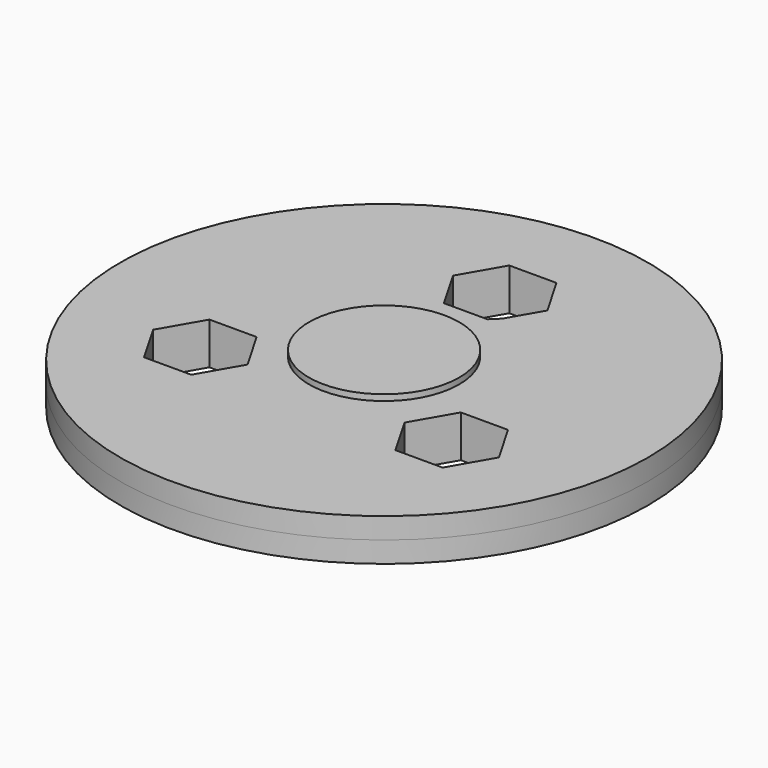
from build123d import *

# Parameters (mm, degrees)
F0_R           = 12.5
F0_R_2         = 11.1
F1_DEPTH       = 1.5
F2_DEPTH       = 3.5
F0_R_3         = 4
F3_DEPTH       = 3.5
F4_START       = 3.5
F0_R_4         = 7.5
F4_DEPTH       = 0.5
F5_START       = 4
F5_DEPTH       = 1
F8_R           = 2.5702688947
F8_R_2         = 2.6203971893
F8_R_3         = 1.9967906643
F8_R_4         = 1.9017675277
F9_DEPTH       = 0.25
F7_TEXT_SIZE   = 4.6829839388
F10_DEPTH      = 0.25
F12_DEPTH      = 3.5
F12_DEPTH_BACK = 3.5
F14_DEPTH      = 3.5
F14_DEPTH_BACK = 3.5
F16_DEPTH      = 3.5
F16_DEPTH_BACK = 3.5
F17_R          = 70.1541780483
F17_R_2        = 43.9177935103
F18_DEPTH      = 25
F18_DEPTH_BACK = 25


# Not quite as in the source:
# - Text() gives the source's letters only with a copy of the font that has no kerning and outlines rounded to 1/6400 em; it was checked with that copy


with BuildPart() as f1:
    # F0 (on Top) → F1 (new body, symmetric)
    with BuildSketch(Plane.XY):
        with BuildLine():
            ThreePointArc((-3.1128243989, 13.7521025397), (-7.595688921, 11.879204932), (-11.1767513589, 8.5959425929))
            ThreePointArc((-11.1767513589, 8.5959425929), (-12.2109581934, 7.05), (-13.0326803344, 5.3813793122))
            ThreePointArc((-13.0326803344, 5.3813793122), (-14.0855377083, 0.6384570988), (-13.4660823543, -4.1802662628))
            ThreePointArc((-13.4660823543, -4.1802662628), (-17.4115804876, -1.8023831124), (-21.9880010034, -1.2754494733))
            ThreePointArc((-21.9880010034, -1.2754494733), (-30.3108891325, -17.5), (-12.0985721468, -18.4044427108))
            ThreePointArc((-12.0985721468, -18.4044427108), (-10.2666998065, -14.1776794661), (-10.3532579553, -9.5718362768))
            ThreePointArc((-10.3532579553, -9.5718362768), (-6.4898487874, -12.5176620308), (-1.8559289755, -13.9773219051))
            ThreePointArc((-1.8559289755, -13.9773219051), (0, -14.1), (1.8559289755, -13.9773219051))
            ThreePointArc((1.8559289755, -13.9773219051), (6.4898487874, -12.5176620308), (10.3532579553, -9.5718362768))
            ThreePointArc((10.3532579553, -9.5718362768), (10.2666998065, -14.1776794661), (12.0985721468, -18.4044427108))
            ThreePointArc((12.0985721468, -18.4044427108), (30.3108891325, -17.5), (21.9880010034, -1.2754494733))
            ThreePointArc((21.9880010034, -1.2754494733), (17.4115804876, -1.8023831124), (13.4660823543, -4.1802662628))
            ThreePointArc((13.4660823543, -4.1802662628), (14.0855377083, 0.6384570988), (13.0326803344, 5.3813793122))
            ThreePointArc((13.0326803344, 5.3813793122), (12.2109581934, 7.05), (11.1767513589, 8.5959425929))
            ThreePointArc((11.1767513589, 8.5959425929), (7.595688921, 11.879204932), (3.1128243989, 13.7521025397))
            ThreePointArc((3.1128243989, 13.7521025397), (7.1448806811, 15.9800625785), (9.8894288566, 19.6798921841))
            ThreePointArc((9.8894288566, 19.6798921841), (0, 35), (-9.8894288566, 19.6798921841))
            ThreePointArc((-9.8894288566, 19.6798921841), (-7.1448806811, 15.9800625785), (-3.1128243989, 13.7521025397))
        make_face()
        Polygon((-16.9868310906, -5.2740181695), (-13.0608492601, -12.0740181695), (-16.9868310906, -18.8740181695), (-24.8387947516, -18.8740181695), (-28.7647765821, -12.0740181695), (-24.8387947516, -5.2740181695), align=None, mode=Mode.SUBTRACT)
        Circle(F0_R, mode=Mode.SUBTRACT)
        Polygon((13.0608492601, -12.0740181695), (16.9868310906, -5.2740181695), (24.8387947516, -5.2740181695), (28.7647765821, -12.0740181695), (24.8387947516, -18.8740181695), (16.9868310906, -18.8740181695), align=None, mode=Mode.SUBTRACT)
        Polygon((7.851963661, 24.148036339), (3.9259818305, 17.348036339), (-3.9259818305, 17.348036339), (-7.851963661, 24.148036339), (-3.9259818305, 30.948036339), (3.9259818305, 30.948036339), align=None, mode=Mode.SUBTRACT)
        Circle(F0_R)
        Circle(F0_R_2, mode=Mode.SUBTRACT)
        with BuildLine():
            ThreePointArc((-13.4660823543, -4.1802662628), (-14.0855377083, 0.6384570988), (-13.0326803344, 5.3813793122))
            ThreePointArc((-13.0326803344, 5.3813793122), (-16.589205157, 0.8137766881), (-21.9880010034, -1.2754494733))
            ThreePointArc((-21.9880010034, -1.2754494733), (-17.4115804876, -1.8023831124), (-13.4660823543, -4.1802662628))
        make_face()
        with BuildLine():
            ThreePointArc((-9.8894288566, 19.6798921841), (-8.9993538634, 13.9597847505), (-11.1767513589, 8.5959425929))
            ThreePointArc((-11.1767513589, 8.5959425929), (-7.595688921, 11.879204932), (-3.1128243989, 13.7521025397))
            ThreePointArc((-3.1128243989, 13.7521025397), (-7.1448806811, 15.9800625785), (-9.8894288566, 19.6798921841))
        make_face()
        with BuildLine():
            ThreePointArc((-10.3532579553, -9.5718362768), (-10.2666998065, -14.1776794661), (-12.0985721468, -18.4044427108))
            ThreePointArc((-12.0985721468, -18.4044427108), (-7.5898512936, -14.7735614386), (-1.8559289755, -13.9773219051))
            ThreePointArc((-1.8559289755, -13.9773219051), (-6.4898487874, -12.5176620308), (-10.3532579553, -9.5718362768))
        make_face()
        with BuildLine():
            ThreePointArc((21.9880010034, -1.2754494733), (16.589205157, 0.8137766881), (13.0326803344, 5.3813793122))
            ThreePointArc((13.0326803344, 5.3813793122), (14.0855377083, 0.6384570988), (13.4660823543, -4.1802662628))
            ThreePointArc((13.4660823543, -4.1802662628), (17.4115804876, -1.8023831124), (21.9880010034, -1.2754494733))
        make_face()
        with BuildLine():
            ThreePointArc((10.3532579553, -9.5718362768), (6.4898487874, -12.5176620308), (1.8559289755, -13.9773219051))
            ThreePointArc((1.8559289755, -13.9773219051), (7.5898512936, -14.7735614386), (12.0985721468, -18.4044427108))
            ThreePointArc((12.0985721468, -18.4044427108), (10.2666998065, -14.1776794661), (10.3532579553, -9.5718362768))
        make_face()
        with BuildLine():
            ThreePointArc((11.1767513589, 8.5959425929), (8.9993538634, 13.9597847505), (9.8894288566, 19.6798921841))
            ThreePointArc((9.8894288566, 19.6798921841), (7.1448806811, 15.9800625785), (3.1128243989, 13.7521025397))
            ThreePointArc((3.1128243989, 13.7521025397), (7.595688921, 11.879204932), (11.1767513589, 8.5959425929))
        make_face()
    extrude(amount=F1_DEPTH, both=True)

    # F0 (on Top) → F2 (join, symmetric)
    with BuildSketch(Plane.XY):
        with BuildLine():
            ThreePointArc((-3.1128243989, 13.7521025397), (-7.595688921, 11.879204932), (-11.1767513589, 8.5959425929))
            ThreePointArc((-11.1767513589, 8.5959425929), (-12.2109581934, 7.05), (-13.0326803344, 5.3813793122))
            ThreePointArc((-13.0326803344, 5.3813793122), (-14.0855377083, 0.6384570988), (-13.4660823543, -4.1802662628))
            ThreePointArc((-13.4660823543, -4.1802662628), (-17.4115804876, -1.8023831124), (-21.9880010034, -1.2754494733))
            ThreePointArc((-21.9880010034, -1.2754494733), (-30.3108891325, -17.5), (-12.0985721468, -18.4044427108))
            ThreePointArc((-12.0985721468, -18.4044427108), (-10.2666998065, -14.1776794661), (-10.3532579553, -9.5718362768))
            ThreePointArc((-10.3532579553, -9.5718362768), (-6.4898487874, -12.5176620308), (-1.8559289755, -13.9773219051))
            ThreePointArc((-1.8559289755, -13.9773219051), (0, -14.1), (1.8559289755, -13.9773219051))
            ThreePointArc((1.8559289755, -13.9773219051), (6.4898487874, -12.5176620308), (10.3532579553, -9.5718362768))
            ThreePointArc((10.3532579553, -9.5718362768), (10.2666998065, -14.1776794661), (12.0985721468, -18.4044427108))
            ThreePointArc((12.0985721468, -18.4044427108), (30.3108891325, -17.5), (21.9880010034, -1.2754494733))
            ThreePointArc((21.9880010034, -1.2754494733), (17.4115804876, -1.8023831124), (13.4660823543, -4.1802662628))
            ThreePointArc((13.4660823543, -4.1802662628), (14.0855377083, 0.6384570988), (13.0326803344, 5.3813793122))
            ThreePointArc((13.0326803344, 5.3813793122), (12.2109581934, 7.05), (11.1767513589, 8.5959425929))
            ThreePointArc((11.1767513589, 8.5959425929), (7.595688921, 11.879204932), (3.1128243989, 13.7521025397))
            ThreePointArc((3.1128243989, 13.7521025397), (7.1448806811, 15.9800625785), (9.8894288566, 19.6798921841))
            ThreePointArc((9.8894288566, 19.6798921841), (0, 35), (-9.8894288566, 19.6798921841))
            ThreePointArc((-9.8894288566, 19.6798921841), (-7.1448806811, 15.9800625785), (-3.1128243989, 13.7521025397))
        make_face()
        Polygon((-16.9868310906, -5.2740181695), (-13.0608492601, -12.0740181695), (-16.9868310906, -18.8740181695), (-24.8387947516, -18.8740181695), (-28.7647765821, -12.0740181695), (-24.8387947516, -5.2740181695), align=None, mode=Mode.SUBTRACT)
        Circle(F0_R, mode=Mode.SUBTRACT)
        Polygon((13.0608492601, -12.0740181695), (16.9868310906, -5.2740181695), (24.8387947516, -5.2740181695), (28.7647765821, -12.0740181695), (24.8387947516, -18.8740181695), (16.9868310906, -18.8740181695), align=None, mode=Mode.SUBTRACT)
        Polygon((7.851963661, 24.148036339), (3.9259818305, 17.348036339), (-3.9259818305, 17.348036339), (-7.851963661, 24.148036339), (-3.9259818305, 30.948036339), (3.9259818305, 30.948036339), align=None, mode=Mode.SUBTRACT)
        Circle(F0_R)
        Circle(F0_R_2, mode=Mode.SUBTRACT)
    extrude(amount=F2_DEPTH, both=True)

    # F11 (on Top) → F12 (join, two sides)
    with BuildSketch(Plane.XY) as f12_sk:
        with BuildLine():
            add(Edge.make_bspline(
                [(-15.8134251833, 42.2175228596), (4.602187624, 46.5557886556), (70.8126677862, 64.1511283532), (66.9090925878, -64.3836754274), (-61.3699533575, -75.2487066952), (-52.925858063, 36.4116518926), (-30.1554145734, 39.1698865919), (-15.8134251833, 42.2175228596)],
                knots=[0, 0, 0, 0, 0.1990629664, 0.4216487162, 0.6458388913, 0.8601580575, 1, 1, 1, 1], degree=3))
        make_face()
        with BuildLine():
            add(Edge.make_bspline(
                [(10.4440450668, 24.1399034858), (10.5373756543, 20.9992472694), (6.0290948904, 15.5002209318), (12.8467750766, -1.9247482711), (17.8310075444, 0.1757999553), (25.9497260601, 1.9852096372), (32.0064980869, -10.4180468568), (31.4185675585, -20.0521719521), (23.8027182873, -20.9500376192), (13.4103785354, -20.4456429805), (12.1782729933, -15.9678191409), (8.0744804894, -12.1586400077), (0.1858323264, -13.89079873), (-11.8587270107, -11.3974146146), (-13.3906107199, -20.9523611954), (-27.136369501, -22.6711460325), (-31.3693811374, -11.3314011229), (-26.7750796326, -2.3895006534), (-14.854258176, -2.288776324), (-4.2587101773, 14.1442439273), (-12.0838201734, 23.3267233429), (-5.2347638972, 33.739818418), (-0.0316080083, 32.2430822073), (6.6392421526, 33.8817233612), (10.3533747875, 27.1910379982), (10.4440450668, 24.1399034858)],
                knots=[0, 0, 0, 0, 0.0465076205, 0.1050097771, 0.1345089104, 0.173411209, 0.2258951257, 0.2684048638, 0.306789347, 0.3530522297, 0.3824884269, 0.4146910543, 0.4570473471, 0.5051414763, 0.5451965636, 0.5937425435, 0.6405531277, 0.6834034872, 0.7324508753, 0.7925428623, 0.8401592731, 0.8862933213, 0.9186649995, 0.9548180392, 1, 1, 1, 1], degree=3))
        make_face(mode=Mode.SUBTRACT)
    extrude(amount=F12_DEPTH)
    extrude(f12_sk.sketch, amount=-F12_DEPTH_BACK)

    # F13 (on Top) → F14 (join, two sides)
    with BuildSketch(Plane.XY) as f14_sk:
        with BuildLine():
            add(Edge.make_bspline(
                [(-25.0858962536, 0), (-24.2659789572, 10.4031696784), (-22.6809452802, 30.5142161314), (2.7718626418, 5.4457263415), (15.3121114709, 46.0786693707), (48.7483758652, -1.349138396), (40.9309414604, -14.8384270596), (37.6365184784, -20.5231234431)],
                knots=[0, 0, 0, 0, 0.191099643, 0.3694271047, 0.5609504055, 0.8149747169, 1, 1, 1, 1], degree=3))
            add(Edge.make_bspline(
                [(-25.0858962536, 0), (-20.6627527559, -1.1678259648), (-11.9575106455, -3.4662393806), (-13.6861794035, -17.2090995637), (-0.3870514271, -25.1532853823), (9.1750335046, -23.6737132537), (11.4993654913, -9.5381163419), (15.4857406669, -2.5354470572), (30.103390425, -3.0709259889), (33.0794347123, -15.1834302125), (20.4033026888, -22.6783054437), (31.4974949251, -21.2908326896), (37.6365184784, -20.5231234431)],
                knots=[0, 0, 0, 0, 0.106139805, 0.2088950739, 0.3228310232, 0.4084912182, 0.5192133822, 0.6033268526, 0.7089617928, 0.8043206387, 0.8917208298, 1, 1, 1, 1], degree=3))
        make_face()
        with BuildLine():
            add(Edge.make_bspline(
                [(-13.1227970123, 7.7634528279), (-14.8565072208, 4.8849996374), (-10.3160175365, -5.2885200643), (-1.223188243, -22.0551348459), (14.1477919362, -5.1802593214), (11.1072608598, -0.4103655322), (14.6017629157, 9.5444494043), (-0.0170075222, 12.2147370021), (-11.3705839059, 10.6726261038), (-13.1227970123, 7.7634528279)],
                knots=[0, 0, 0, 0, 0.1535046532, 0.3150136102, 0.4839325326, 0.579912713, 0.6954216068, 0.8448570794, 1, 1, 1, 1], degree=3))
        make_face(mode=Mode.SUBTRACT)
    extrude(amount=F14_DEPTH)
    extrude(f14_sk.sketch, amount=-F14_DEPTH_BACK)

    # F15 (on Top) → F16 (join, two sides)
    with BuildSketch(Plane.XY) as f16_sk:
        with BuildLine():
            add(Edge.make_bspline(
                [(2.6121865958, -14.2520507798), (2.8577335579, -15.9643788276), (10.3218108858, -17.6159644372), (9.5897241742, -7.1874142222), (2.3499542827, -12.4233670082), (2.6121865958, -14.2520507798)],
                knots=[0, 0, 0, 0, 0.3339633441, 0.6433432551, 1, 1, 1, 1], degree=3))
        make_face()
    extrude(amount=F16_DEPTH)
    extrude(f16_sk.sketch, amount=-F16_DEPTH_BACK)

    # F17 (on Top) → F18 (cut, two sides)
    with BuildSketch(Plane.XY) as f18_sk:
        Circle(F17_R)
        Circle(F17_R_2, mode=Mode.SUBTRACT)
    extrude(amount=-F18_DEPTH, mode=Mode.SUBTRACT)
    extrude(f18_sk.sketch, amount=F18_DEPTH_BACK, mode=Mode.SUBTRACT)


with BuildPart() as f3:
    # F0 (on Top) → F3 (new body)
    with BuildSketch(Plane.XY):
        Circle(F0_R_3)
    extrude(amount=F3_DEPTH)

    # F0 (on Top) → F4 (join)
    with BuildSketch(Plane.XY.offset(F4_START)):
        Circle(F0_R_4)
        Circle(F0_R_3, mode=Mode.SUBTRACT)
        Circle(F0_R_3)
    extrude(amount=F4_DEPTH)

    # F0 (on Top) → F5 (join)
    with BuildSketch(Plane.XY.offset(F5_START)):
        Circle(F0_R)
        Circle(F0_R_2, mode=Mode.SUBTRACT)
        Circle(F0_R_2)
        Circle(F0_R_4, mode=Mode.SUBTRACT)
        Circle(F0_R_4)
        Circle(F0_R_3, mode=Mode.SUBTRACT)
        Circle(F0_R_3)
    extrude(amount=F5_DEPTH)


with BuildPart() as f6_1:
    # F6: instance of F3
    add(f3.part.mirror(Plane(origin=(0, 0, 0), x_dir=(1, 0, 0), z_dir=(0, 0, -1))))

    # F8 (on face) → F9 (cut)
    with BuildSketch(Plane(origin=(0, 0, -5), x_dir=(1, 0, 0), z_dir=(0, 0, -1))):
        with BuildLine():
            add(Edge.make_bspline(
                [(-0.096452734, 6.1445777375), (-0.0602709809, 6.289685204), (0.0044720735, 6.5493378215), (0.0304961839, 6.3405444376), (0.0419766693, 6.2484352694)],
                knots=[0, 0, 0, 0, 0.5588512882, 1, 1, 1, 1], degree=3))
            ThreePointArc((0.0419766693, 6.2484352694), (6.5545094926, 6.6656830815), (0.0918355037, 7.571787062))
            add(Edge.make_bspline(
                [(-0.0746485587, 7.6168120207), (-0.0501907607, 7.4626956429), (-0.0029108972, 7.164770679), (0.0491340277, 7.5470012931), (0.0918355037, 7.571787062)],
                knots=[0, 0, 0, 0, 0.1822855952, 0.3523796555, 0.3523796555, 0.3523796555, 0.3523796555], degree=3))
            ThreePointArc((-0.0746485587, 7.6168120207), (-6.4457158602, 6.9748905916), (-0.096452734, 6.1445777375))
        make_face()
        with Locations((-3.2230346393, 6.9271618387)):
            Circle(F8_R, mode=Mode.SUBTRACT)
        with Locations((3.2769653607, 6.7891684093)):
            Circle(F8_R_2, mode=Mode.SUBTRACT)
        with Locations((3.2769653607, 6.7891684093)):
            Circle(F8_R_3)
        with Locations((-3.2230346393, 6.9271618387)):
            Circle(F8_R_4)
    extrude(amount=-F9_DEPTH, mode=Mode.SUBTRACT)

    # F7 (on face) → F10 (cut)
    with BuildSketch(Plane(origin=(0, 0, -5), x_dir=(1, 0, 0), z_dir=(0, 0, -1))):
        with Locations((-10, -1.5)):
            Text('<~Alex~>', F7_TEXT_SIZE, font='Open Sans', text_align=(TextAlign.LEFT, TextAlign.BOTTOM))
    extrude(amount=-F10_DEPTH, mode=Mode.SUBTRACT)


solid = Compound([f1.part, f3.part, f6_1.part])
